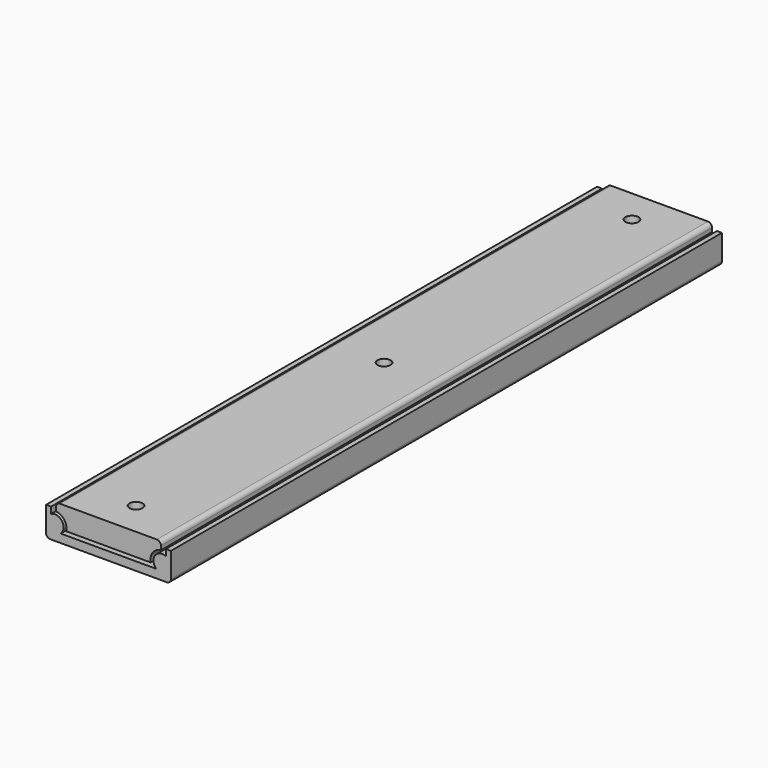
from build123d import *

# Parameters (mm, degrees)
F1_DEPTH      = 254
F2_R          = 2.413
F3_DEPTH      = 386
F3_DEPTH_BACK = 12.701


# Not quite as in the source:
# - an extrude ends at something that could not be found from the text; its depth is read off the source's solid


with BuildPart() as f1:
    # F0 (on Front) → F1 (new body)
    with BuildSketch(Plane.XZ):
        with BuildLine():
            Line((-21.180855953, 10.6905996799), (-23.01875, 10.6905996799))
            Line((-23.01875, 10.6905996799), (-23.01875, 1.524))
            ThreePointArc((-23.01875, 1.524), (-22.5723807345, 0.4463692655), (-21.49475, 0))
            Line((-21.49475, 0), (21.49475, 0))
            ThreePointArc((21.49475, 0), (22.5723807345, 0.4463692655), (23.01875, 1.524))
            Line((23.01875, 1.524), (23.01875, 10.6905996799))
            Line((23.01875, 10.6905996799), (21.180855953, 10.6905996799))
            Line((21.180855953, 10.6905996799), (21.180855953, 8.3211223024))
            ThreePointArc((21.180855953, 8.3211223024), (17.1238073852, 7.2644445689), (17.6117553886, 3.1005380306))
            Line((17.6117553886, 3.1005380306), (-17.6117553886, 3.1005380306))
            ThreePointArc((-17.6117553886, 3.1005380306), (-17.1238073852, 7.2644445689), (-21.180855953, 8.3211223024))
            Line((-21.180855953, 8.3211223024), (-21.180855953, 10.6905996799))
        make_face()
    extrude(amount=F1_DEPTH)


with BuildPart() as f1b:
    # F0 (on Front) → F1, piece 2 (new body)
    with BuildSketch(Plane.XZ):
        with BuildLine():
            ThreePointArc((-19.3494111094, 9.7232580064), (-16.2862756718, 7.9644871947), (-15.5882310877, 4.5020014929))
            Line((-15.5882310877, 4.5020014929), (15.5882310877, 4.5020014929))
            ThreePointArc((15.5882310877, 4.5020014929), (16.2862756718, 7.9644871947), (19.3494111094, 9.7232580064))
            Line((19.3494111094, 9.7232580064), (19.3494111094, 11.176))
            ThreePointArc((19.3494111094, 11.176), (18.9030418439, 12.2536307345), (17.8254111094, 12.7))
            Line((17.8254111094, 12.7), (-17.8254111094, 12.7))
            ThreePointArc((-17.8254111094, 12.7), (-18.9030418439, 12.2536307345), (-19.3494111094, 11.176))
            Line((-19.3494111094, 11.176), (-19.3494111094, 9.7232580064))
        make_face()
    extrude(amount=F1_DEPTH)


with BuildPart() as f3_tool:
    # F2 (on Top) → F3 (new body, two sides)
    with BuildSketch(Plane.XY) as f3_sk:
        with Locations((0, -12.7)):
            Circle(F2_R)
        with Locations((0, -127)):
            Circle(F2_R)
        with Locations((0, -241.3)):
            Circle(F2_R)
    extrude(amount=-F3_DEPTH)
    extrude(f3_sk.sketch, amount=F3_DEPTH_BACK)


with BuildPart() as f1_1:
    add(f1.part)

    # F3: cut by f3_tool
    add(f3_tool.part, mode=Mode.SUBTRACT)


with BuildPart() as f1b_1:
    add(f1b.part)

    # F3: cut by f3_tool
    add(f3_tool.part, mode=Mode.SUBTRACT)


solid = Compound([f1_1.part, f1b_1.part])
